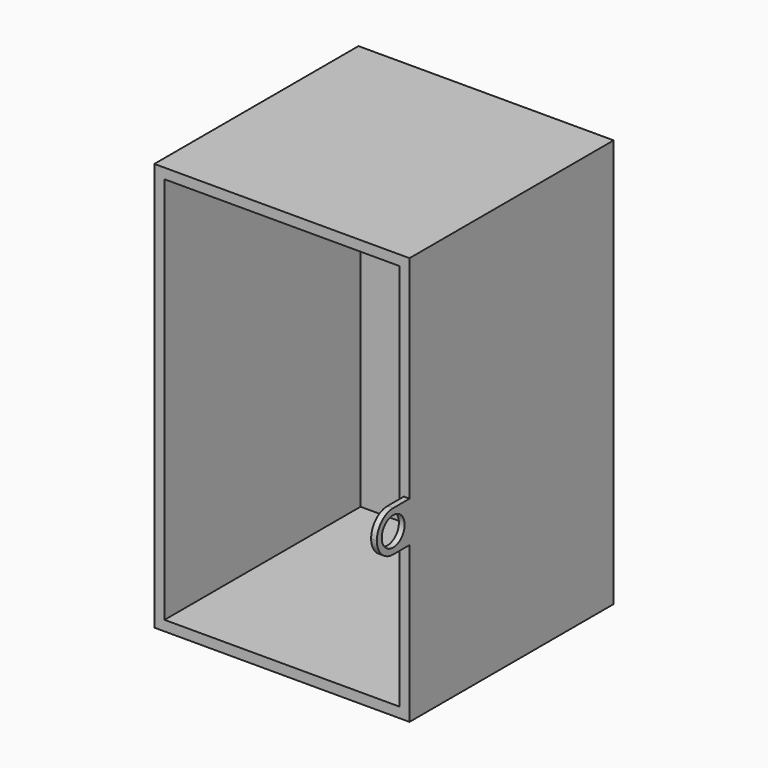
from build123d import *

# Parameters (mm, degrees)
F0_W     = 79.375
F0_H     = 127
F1_DEPTH = 3.175
F2_W     = 73.025
F2_H     = 3.175
F3_DEPTH = 76.2
F4_W     = 1.778
F4_H     = 12.7
F5_DEPTH = 12.7
F6_R     = 6.35
F7_R     = 6.34999
F8_R     = 4.445
F9_DEPTH = 25.4


# Not quite as in the source:
# - a fillet or chamfer is up to 0.001 mm smaller than in the source, because OpenCascade refuses the exact size


with BuildPart() as f1:
    # F0 (on Front) → F1 (new body)
    with BuildSketch(Plane.XZ):
        with Locations((-10.1727880716, 3.2072235078)):
            Rectangle(F0_W, F0_H)
    extrude(amount=F1_DEPTH)

    # F2 (on face) → F3 (join)
    with BuildSketch(Plane.XZ.offset(3.175)):
        Polygon((-46.6852880716, 63.5322235078), (-46.6852880716, 66.7072235078), (-49.8602880716, 66.7072235078), (-49.8602880716, -60.2927764922), (-46.6852880716, -60.2927764922), (-46.6852880716, -57.1177764922), align=None)
        with Locations((-10.1727880716, 65.1197235078)):
            Rectangle(F2_W, F2_H)
        Polygon((29.5147119284, 66.7072235078), (26.3397119284, 66.7072235078), (26.3397119284, 63.5322235078), (26.3397119284, -57.1177764922), (26.3397119284, -60.2927764922), (29.5147119284, -60.2927764922), align=None)
        with Locations((-10.1727880716, -58.7052764922)):
            Rectangle(F2_W, F2_H)
    extrude(amount=F3_DEPTH)

    # F4 (on face) → F5 (join)
    with BuildSketch(Plane.XZ.offset(79.375)):
        with Locations((28.6257119284, -5.5081006922)):
            Rectangle(F4_W, F4_H)
    extrude(amount=F5_DEPTH)

    # F6
    f6_edges = [f1.edges().sort_by_distance(p)[0] for p in [
        (28.625712, -92.075, 0.841899),
    ]]
    fillet(f6_edges, radius=F6_R)

    # F7 (radius 6.35 in the source; OpenCascade refuses exactly that, so slightly less here)
    f7_edges = [f1.edges().sort_by_distance(p)[0] for p in [
        (28.625712, -92.075, -11.858101),
    ]]
    fillet(f7_edges, radius=F7_R)

    # F8 (on face) → F9 (cut)
    with BuildSketch(Plane.YZ.offset(29.5147119284)):
        with Locations((-85.725, -5.5081006922)):
            Circle(F8_R)
    extrude(amount=-F9_DEPTH, mode=Mode.SUBTRACT)


solid = f1.part
